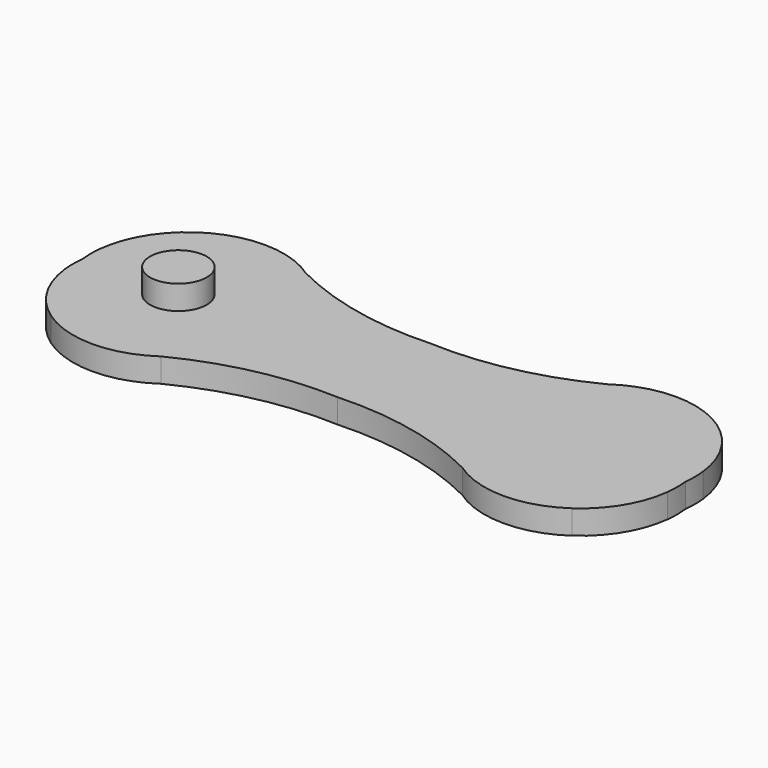
from build123d import *

# Parameters (mm, degrees)
F1_DEPTH = 2
F2_DEPTH = 4


with BuildPart() as f1:
    # F0 (on Top) → F1 (new body)
    with BuildSketch(Plane.XY):
        with BuildLine():
            ThreePointArc((18.0739206718, 6.0497422268), (13.5205869532, 7.4719650911), (8.9672532347, 6.0497422268))
            Line((8.9672532347, 6.0497422268), (18.0739206718, 6.0497422268))
        make_face()
        with BuildLine():
            Line((18.0739206718, 6.0497422268), (8.9672532347, 6.0497422268))
            ThreePointArc((8.9672532347, 6.0497422268), (2.8913578077, 3.8979685049), (-3.5327467653, 3.3711707982))
            Line((-3.5327467653, 3.3711707982), (-3.5327467653, -1.4502577732))
            Line((-3.5327467653, -1.4502577732), (21.4672532347, -1.4502577732))
            Line((21.4672532347, -1.4502577732), (21.4672532347, 0.3941879553))
            ThreePointArc((21.4672532347, 0.3941879553), (20.3805303589, 3.5879311345), (18.0739206718, 6.0497422268))
        make_face()
        with BuildLine():
            Line((-3.5327467653, -1.4502577732), (-3.5327467653, 3.3711707982))
            ThreePointArc((-3.5327467653, 3.3711707982), (-9.9568513384, 3.8979685049), (-16.0327467653, 6.0497422268))
            Line((-16.0327467653, 6.0497422268), (-25.1394142025, 6.0497422268))
            ThreePointArc((-25.1394142025, 6.0497422268), (-27.4460238896, 3.5879311345), (-28.5327467653, 0.3941879553))
            Line((-28.5327467653, 0.3941879553), (-28.5327467653, -1.4502577732))
            Line((-28.5327467653, -1.4502577732), (-22.9360804839, -1.4502577732))
            ThreePointArc((-22.9360804839, -1.4502577732), (-20.5860804839, 0.8997422268), (-18.2360804839, -1.4502577732))
            Line((-18.2360804839, -1.4502577732), (-3.5327467653, -1.4502577732))
        make_face()
        with BuildLine():
            Line((-25.1394142025, 6.0497422268), (-16.0327467653, 6.0497422268))
            ThreePointArc((-16.0327467653, 6.0497422268), (-20.5860804839, 7.4719650911), (-25.1394142025, 6.0497422268))
        make_face()
        with BuildLine():
            ThreePointArc((21.4672532347, -1.4502577732), (21.5205869532, -0.5280349089), (21.4672532347, 0.3941879553))
            Line((21.4672532347, 0.3941879553), (21.4672532347, -1.4502577732))
        make_face()
        with BuildLine():
            Line((21.4672532347, -1.4502577732), (-3.5327467653, -1.4502577732))
            Line((-3.5327467653, -1.4502577732), (-3.5327467653, -6.2716863446))
            ThreePointArc((-3.5327467653, -6.2716863446), (2.8913578077, -6.7984840513), (8.9672532347, -8.9502577732))
            Line((8.9672532347, -8.9502577732), (18.0739206718, -8.9502577732))
            ThreePointArc((18.0739206718, -8.9502577732), (20.3805303589, -6.4884466809), (21.4672532347, -3.2947035017))
            Line((21.4672532347, -3.2947035017), (21.4672532347, -1.4502577732))
        make_face()
        with BuildLine():
            Line((-3.5327467653, -6.2716863446), (-3.5327467653, -1.4502577732))
            Line((-3.5327467653, -1.4502577732), (-18.2360804839, -1.4502577732))
            ThreePointArc((-18.2360804839, -1.4502577732), (-20.5860804839, -3.8002577732), (-22.9360804839, -1.4502577732))
            Line((-22.9360804839, -1.4502577732), (-28.5327467653, -1.4502577732))
            Line((-28.5327467653, -1.4502577732), (-28.5327467653, -3.2947035017))
            ThreePointArc((-28.5327467653, -3.2947035017), (-27.4460238896, -6.4884466809), (-25.1394142025, -8.9502577732))
            Line((-25.1394142025, -8.9502577732), (-16.0327467653, -8.9502577732))
            ThreePointArc((-16.0327467653, -8.9502577732), (-9.9568513384, -6.7984840513), (-3.5327467653, -6.2716863446))
        make_face()
        with BuildLine():
            ThreePointArc((21.4672532347, -3.2947035017), (21.5205869532, -2.3724806375), (21.4672532347, -1.4502577732))
            Line((21.4672532347, -1.4502577732), (21.4672532347, -3.2947035017))
        make_face()
        with BuildLine():
            Line((-28.5327467653, -1.4502577732), (-28.5327467653, 0.3941879553))
            ThreePointArc((-28.5327467653, 0.3941879553), (-28.5860804839, -0.5280349089), (-28.5327467653, -1.4502577732))
        make_face()
        with BuildLine():
            ThreePointArc((-25.1394142025, -8.9502577732), (-20.5860804839, -10.3724806375), (-16.0327467653, -8.9502577732))
            Line((-16.0327467653, -8.9502577732), (-25.1394142025, -8.9502577732))
        make_face()
        with BuildLine():
            Line((18.0739206718, -8.9502577732), (8.9672532347, -8.9502577732))
            ThreePointArc((8.9672532347, -8.9502577732), (13.5205869532, -10.3724806375), (18.0739206718, -8.9502577732))
        make_face()
        with BuildLine():
            Line((-28.5327467653, -3.2947035017), (-28.5327467653, -1.4502577732))
            ThreePointArc((-28.5327467653, -1.4502577732), (-28.5860804839, -2.3724806375), (-28.5327467653, -3.2947035017))
        make_face()
    extrude(amount=F1_DEPTH)

    # F0 (on Top) → F2 (join)
    with BuildSketch(Plane.XY):
        with BuildLine():
            ThreePointArc((-22.9360804839, -1.4502577732), (-20.5860804839, -3.8002577732), (-18.2360804839, -1.4502577732))
            Line((-18.2360804839, -1.4502577732), (-20.5860804839, -1.4502577732))
            Line((-20.5860804839, -1.4502577732), (-22.9360804839, -1.4502577732))
        make_face()
        with BuildLine():
            Line((-20.5860804839, -1.4502577732), (-18.2360804839, -1.4502577732))
            ThreePointArc((-18.2360804839, -1.4502577732), (-20.5860804839, 0.8997422268), (-22.9360804839, -1.4502577732))
            Line((-22.9360804839, -1.4502577732), (-20.5860804839, -1.4502577732))
        make_face()
    extrude(amount=F2_DEPTH)


solid = f1.part
